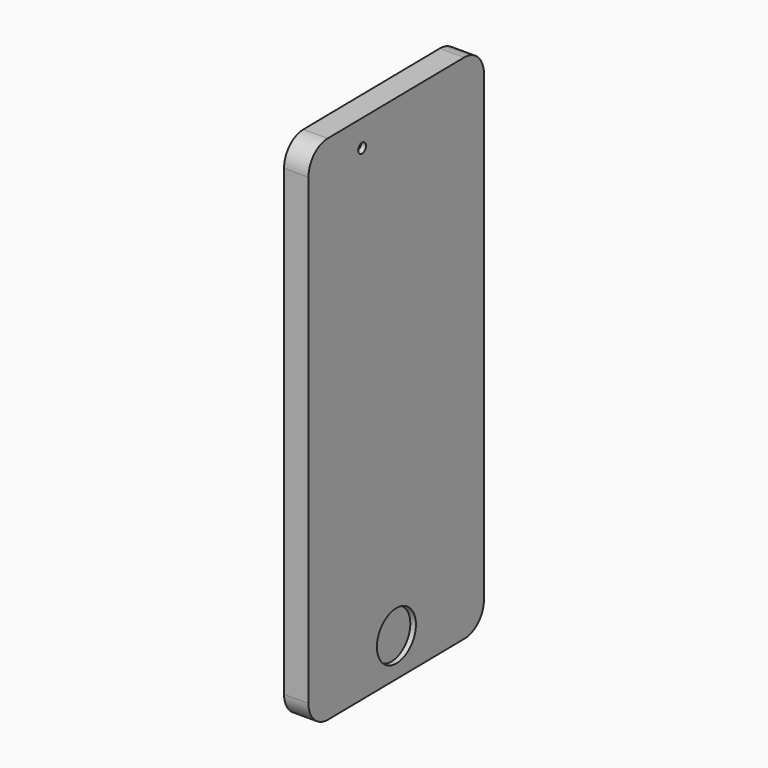
from build123d import *

# Parameters (mm, degrees)
F0_R     = 6.35
F0_R_2   = 1.27
F1_DEPTH = 6.35
F2_R     = 6.1829946026
F3_DEPTH = 5.08
F2_R_2   = 1.27


# Not quite as in the source:
# - a feature of the source that left no trace in its solid (it failed there, or was rolled back) is left out


with BuildPart() as f1:
    # F0 (on Right) → F1 (new body)
    with BuildSketch(Plane.YZ):
        with BuildLine():
            Line((17.2854172051, -77.1269578294), (17.2854172051, 43.5222112587))
            ThreePointArc((17.2854172051, 43.5222112587), (15.3997912282, 48.0379464793), (10.8627826911, 49.87179583))
            Line((10.8627826911, 49.87179583), (-33.5834784501, 49.3633637362))
            ThreePointArc((-33.5834784501, 49.3633637362), (-38.0265791567, 47.4781531881), (-39.8608439361, 43.013779165))
            Line((-39.8608439361, 43.013779165), (-39.8608439361, -77.6353899231))
            ThreePointArc((-39.8608439361, -77.6353899231), (-37.9752179592, -82.1511251437), (-33.4382094221, -83.9849744944))
            Line((-33.4382094221, -83.9849744944), (11.0080517191, -83.4765424006))
            ThreePointArc((11.0080517191, -83.4765424006), (15.4511524256, -81.5913318525), (17.2854172051, -77.1269578294))
        make_face()
        with Locations((-11.2150788515, -73.7819895148)):
            Circle(F0_R, mode=Mode.SUBTRACT)
        with Locations((-22.3856065422, 42.5772145391)):
            Circle(F0_R_2, mode=Mode.SUBTRACT)
    extrude(amount=F1_DEPTH)


with BuildPart() as f3:
    # F2 (on Right) → F3 (new body)
    with BuildSketch(Plane.YZ):
        with Locations((-11.2779513001, -73.9273875952)):
            Circle(F2_R)
    extrude(amount=F3_DEPTH)


with BuildPart() as f3b:
    # F2 (on Right) → F3, piece 2 (new body)
    with BuildSketch(Plane.YZ):
        with Locations((-22.4166736007, 42.7506938577)):
            Circle(F2_R_2)
    extrude(amount=F3_DEPTH)


solid = Compound([f1.part, f3.part, f3b.part])
